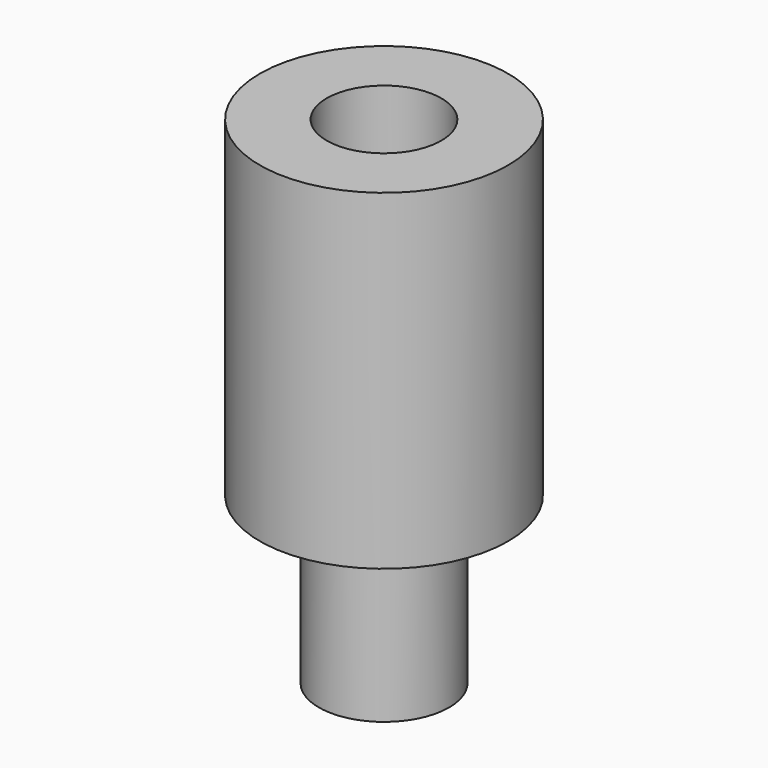
from build123d import *

# Parameters (mm, degrees)
F0_R     = 9.525
F0_R_2   = 5
F1_DEPTH = 25.4
F2_DEPTH = 12.7
F4_D     = 8.8
F4_DEPTH = 19.05
F4_TIP   = 2.6437867237


with BuildPart() as f1:
    # F0 (on Top) → F1 (new body)
    with BuildSketch(Plane.XY):
        Circle(F0_R)
        Circle(F0_R_2, mode=Mode.SUBTRACT)
        Circle(F0_R_2)
    extrude(amount=F1_DEPTH)

    # F0 (on Top) → F2 (join)
    with BuildSketch(Plane.XY):
        Circle(F0_R_2)
    extrude(amount=-F2_DEPTH)

    # F4
    with Locations(Plane.XY.offset(25.4)):
        with Locations((0, 0)):
            Hole(F4_D / 2, depth=F4_DEPTH)
            with Locations((0, 0, -(F4_DEPTH + F4_TIP / 2))):  # 118° drill point
                Cone(0, F4_D / 2, F4_TIP, mode=Mode.SUBTRACT)


solid = f1.part
